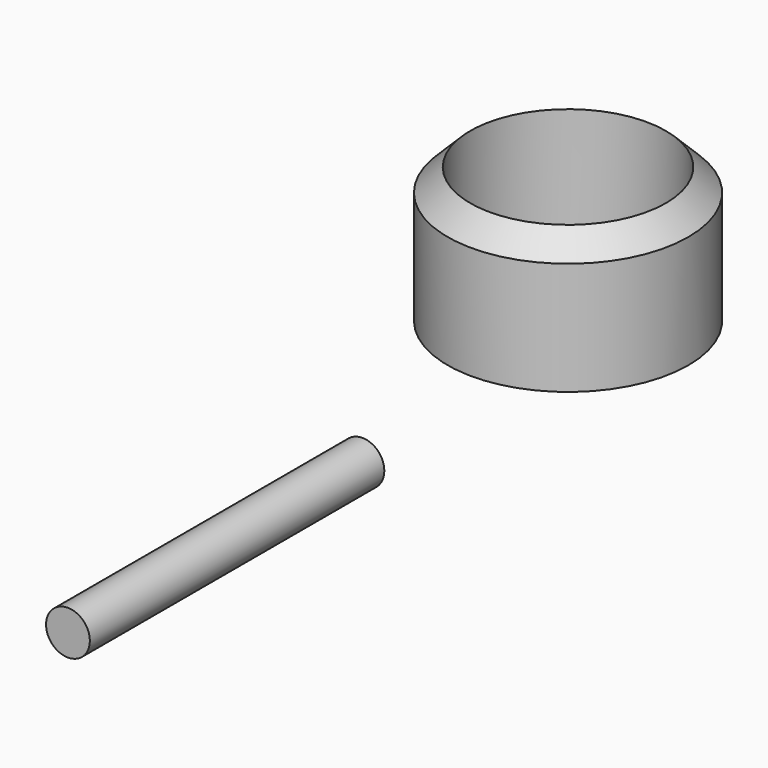
from build123d import *

# Parameters (mm, degrees)
F0_R     = 39.9760214069
F0_R_2   = 32.4968914301
F1_DEPTH = 45.1091602445
F3_R     = 7.2748439962
F4_DEPTH = 122.2406476736


# Not quite as in the source:
# - a fillet or chamfer that OpenCascade refuses, or shapes differently, is made with other operations: its cross-section is extruded or revolved along the edge and cut away or added


with BuildPart() as f1:
    # F0 (on Top) → F1 (new body)
    with BuildSketch(Plane.XY):
        with Locations((0, 51.2107610703)):
            Circle(F0_R)
        with Locations((0, 51.2107610703)):
            Circle(F0_R_2, mode=Mode.SUBTRACT)
    extrude(amount=F1_DEPTH)

    # F2: chamfer of 7.62 on 1 edges, made by hand

    # F2_s1 → F2_t2 (revolve, cut)
    with BuildSketch(Plane.XZ.offset(-51.2107610703)):
        Polygon((39.9760214069, 37.4891602445), (32.3560214069, 45.1091602445), (39.9760214069, 45.1091602445), align=None)
    revolve(axis=Axis((0, 51.2107610703, 45.1091602445), (0, 0, 1)), mode=Mode.SUBTRACT)


with BuildPart() as f4:
    # F3 (on Front) → F4 (new body)
    with BuildSketch(Plane.XZ):
        with Locations((-27.3221582174, -29.5520946383)):
            Circle(F3_R)
    extrude(amount=F4_DEPTH)


solid = Compound([f1.part, f4.part])
